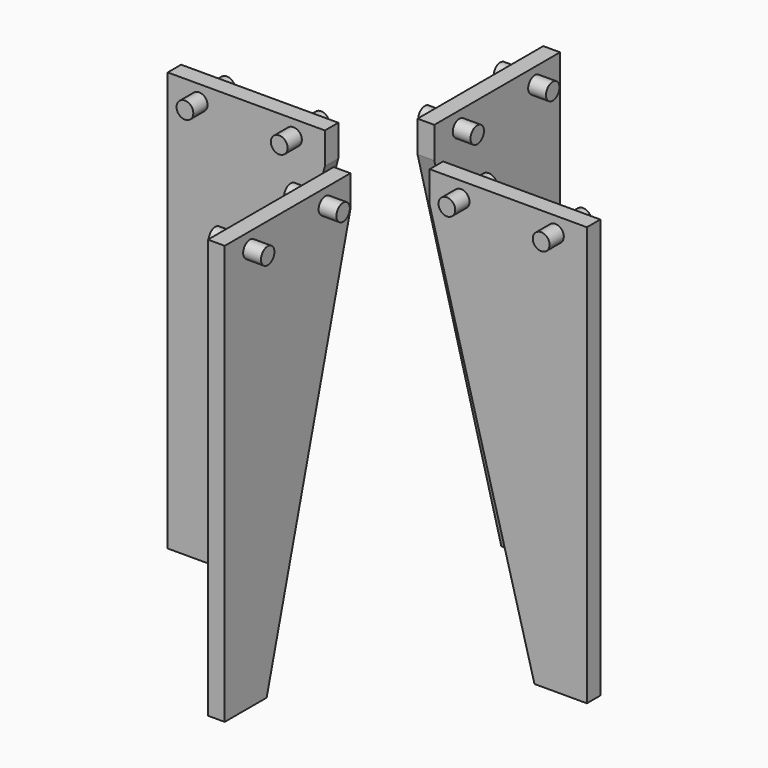
from build123d import *

# Parameters (mm, degrees)
F0_R     = 8
F1_DEPTH = 8
F2_DEPTH = 25
F3_R     = 8
F4_DEPTH = 33.001
F5_COUNT = 4
F5_ANGLE = 270


with BuildPart() as f1:
    # F0 (on Front) → F1 (new body, symmetric)
    with BuildSketch(Plane.XZ):
        Polygon((-50, 370), (-50, 400), (-200, 400), (-200, 0), (-150, 0), align=None)
        with Locations((-170, 385)):
            Circle(F0_R, mode=Mode.SUBTRACT)
        with Locations((-80, 385)):
            Circle(F0_R, mode=Mode.SUBTRACT)
        with Locations((-80, 385)):
            Circle(F0_R)
        with Locations((-170, 385)):
            Circle(F0_R)
    extrude(amount=F1_DEPTH, both=True)

    # F3 (on face) → F4 (cut, through all)
    with BuildSketch(Plane.XZ.offset(8)):
        with Locations((-170, 385)):
            Circle(F3_R)
        with Locations((-80, 385)):
            Circle(F3_R)
    extrude(amount=-F4_DEPTH, mode=Mode.SUBTRACT)


with BuildPart() as f2:
    # F0 (on Front) → F2 (new body, symmetric)
    with BuildSketch(Plane.XZ):
        with Locations((-80, 385)):
            Circle(F0_R)
    extrude(amount=F2_DEPTH, both=True)


with BuildPart() as f2b:
    # F0 (on Front) → F2, piece 2 (new body, symmetric)
    with BuildSketch(Plane.XZ):
        with Locations((-170, 385)):
            Circle(F0_R)
    extrude(amount=F2_DEPTH, both=True)


with BuildPart() as f5_1:
    # F5: instance of F1
    add(f1.part.rotate(Axis((0, 0, 159.6400429041), (0, 0, 1)), 1 * F5_ANGLE / (F5_COUNT - 1)))


with BuildPart() as f5_2:
    # F5: instance of F1
    add(f1.part.rotate(Axis((0, 0, 159.6400429041), (0, 0, 1)), 2 * F5_ANGLE / (F5_COUNT - 1)))


with BuildPart() as f5_3:
    # F5: instance of F1
    add(f1.part.rotate(Axis((0, 0, 159.6400429041), (0, 0, 1)), 3 * F5_ANGLE / (F5_COUNT - 1)))


with BuildPart() as f5_4:
    # F5: instance of F2
    add(f2.part.rotate(Axis((0, 0, 159.6400429041), (0, 0, 1)), 1 * F5_ANGLE / (F5_COUNT - 1)))


with BuildPart() as f5_5:
    # F5: instance of F2
    add(f2.part.rotate(Axis((0, 0, 159.6400429041), (0, 0, 1)), 2 * F5_ANGLE / (F5_COUNT - 1)))


with BuildPart() as f5_6:
    # F5: instance of F2
    add(f2.part.rotate(Axis((0, 0, 159.6400429041), (0, 0, 1)), 3 * F5_ANGLE / (F5_COUNT - 1)))


with BuildPart() as f5_7:
    # F5: instance of F2b
    add(f2b.part.rotate(Axis((0, 0, 159.6400429041), (0, 0, 1)), 1 * F5_ANGLE / (F5_COUNT - 1)))


with BuildPart() as f5_8:
    # F5: instance of F2b
    add(f2b.part.rotate(Axis((0, 0, 159.6400429041), (0, 0, 1)), 2 * F5_ANGLE / (F5_COUNT - 1)))


with BuildPart() as f5_9:
    # F5: instance of F2b
    add(f2b.part.rotate(Axis((0, 0, 159.6400429041), (0, 0, 1)), 3 * F5_ANGLE / (F5_COUNT - 1)))


solid = Compound([f1.part, f2.part, f2b.part, f5_1.part, f5_2.part, f5_3.part, f5_4.part, f5_5.part, f5_6.part, f5_7.part, f5_8.part, f5_9.part])
